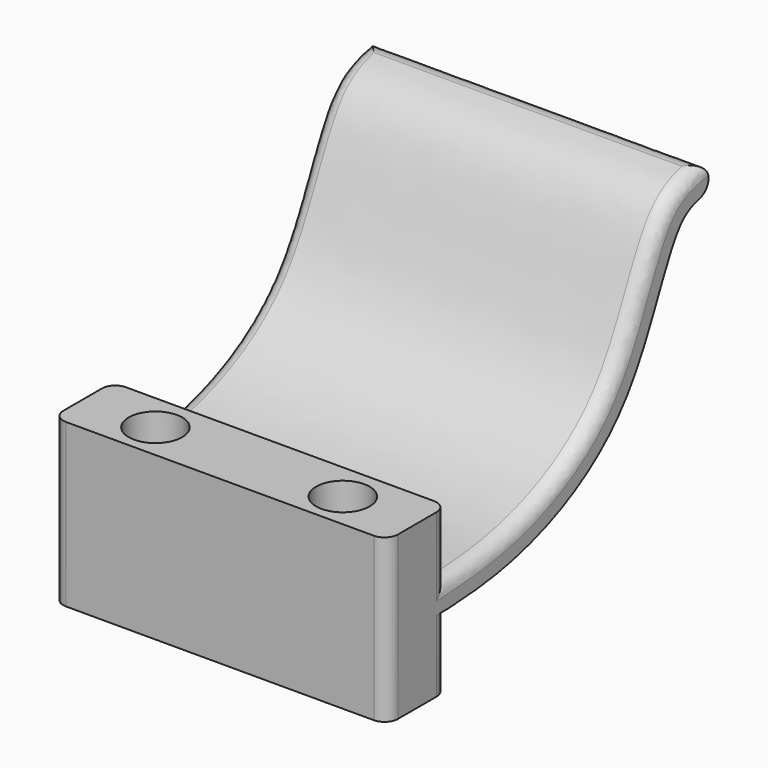
from build123d import *

# Parameters (mm, degrees)
F1_DEPTH       = 25
F3_DEPTH       = 25.001
F5_D           = 3
F5_DEPTH       = 12
F5_CBORE_D     = 4
F5_CBORE_DEPTH = 5
F5_TIP         = 0.9012909285
F6_R           = 1


# Not quite as in the source:
# - ends of sketch curves that miss each other by under 0.0002 mm in the source are joined
# - the dataset's text gives a spline's control points without its knots; the knots are read off the source's solid


with BuildPart() as f1:
    # F0 (on Top) → F1 (new body)
    with BuildSketch(Plane.XY):
        Polygon((12.5, 12.3358736806), (12.5, 15), (10.2798947338, 15), align=None)
        Polygon((12.5, 12.3358736806), (10.2798947338, 15), (7.0256240355, 15), (12.5, 8.4307488427), align=None)
        Polygon((12.5, 8.4307488427), (7.0256240355, 15), (3.7713532076, 15), (12.5, 4.5256238491), align=None)
        Polygon((12.5, 4.5256238491), (3.7713532076, 15), (0.5170825093, 15), (12.5, 0.6204990111), align=None)
        Polygon((12.5, 0.6204990111), (0.5170825093, 15), (-2.7371880471, 15), (12.5, -3.2846256565), align=None)
        Polygon((12.5, -3.2846256565), (-2.7371880471, 15), (-5.9914587454, 15), (12.5, -7.1897504944), align=None)
        Polygon((12.5, -7.1897504944), (-5.9914587454, 15), (-9.2457293017, 15), (12.5, -11.094875162), align=None)
        Polygon((12.5, -11.094875162), (-9.2457293017, 15), (-12.5, 15), (12.5, -15), align=None)
        Polygon((12.5, -15), (-12.5, 15), (-12.5, 11.094875162), (9.2457293017, -15), align=None)
        Polygon((5.9914586034, -15), (-12.5, 7.1897503241), (-12.5, 3.2846254861), (2.7371879051, -15), align=None)
        Polygon((-0.5170827932, -15), (-12.5, -0.6204993518), (-12.5, -4.5256241898), (-3.7713534915, -15), align=None)
        Polygon((-3.7713534915, -15), (-12.5, -4.5256241898), (-12.5, -8.4307490277), (-7.0256241898, -15), align=None)
        Polygon((-7.0256241898, -15), (-12.5, -8.4307490277), (-12.5, -15), align=None)
        Polygon((9.2457293017, -15), (-12.5, 11.094875162), (-12.5, 7.1897503241), (5.9914586034, -15), align=None)
        Polygon((2.7371879051, -15), (-12.5, 3.2846254861), (-12.5, -0.6204993518), (-0.5170827932, -15), align=None)
    extrude(amount=F1_DEPTH)

    # F2 (on face) → F3 (cut, through all)
    with BuildSketch(Plane(origin=(-12.5, 0, 0), x_dir=(0, -1, 0), z_dir=(-1, 0, 0))):
        with BuildLine():
            Line((15, 25), (-15, 25))
            add(Edge.make_bspline(
                [(-15, 25), (-13.5568248924, 24.7224313944), (-9.8278339599, 24.005227496), (-6.8122451266, 12.0375054671), (2.945956356, 7.7369731005), (7.4143120604, 7.46721459), (9.3878423795, 7.3480708525)],
                knots=[0, 0, 0, 0, 0.1895841201, 0.4898625685, 0.7746885533, 1, 1, 1, 1], degree=3))
            Line((9.3878423795, 7.3480708525), (9.3878423795, 12.1319638565))
            Line((9.3878423795, 12.1319638565), (15, 12.1319638565))
            Line((15, 12.1319638565), (15, 25))
        make_face()
        with BuildLine():
            Line((9.3878423795, 0), (9.3878423795, 5.3517055617))
            Line((9.3878423795, 5.3517055617), (9.2673200749, 5.3517055617))
            add(Edge.make_bspline(
                [(-15.0000575165, 22.9623060021), (-14.6750769086, 22.8974842127), (-14.1746868984, 22.789063183), (-13.5954276376, 22.6021711473), (-13.1732029655, 22.4090687875), (-12.867772976, 22.2113862359), (-12.6317224774, 22.0126010766), (-12.4567595118, 21.838250856), (-12.2734281701, 21.6221144569), (-12.0699637563, 21.3450122532), (-11.8562489345, 21.0163300592), (-11.5603798617, 20.5139838197), (-11.176165806, 19.7797133282), (-10.6958775361, 18.767836688), (-10.1906413822, 17.6609048928), (-9.6497850817, 16.4909565123), (-9.0591193515, 15.2873931399), (-8.401307085, 14.0777387133), (-7.7797470029, 13.0871929073), (-7.2259212866, 12.3190564954), (-6.6294247554, 11.5740230358), (-5.8330517423, 10.7238746842), (-4.469813467, 9.5191459149), (-2.6461329718, 8.2928627168), (-0.390600399, 7.2034186589), (1.8283532393, 6.4330776096), (3.8987281726, 5.9261842869), (6.4545278666, 5.5194639384), (8.1724298973, 5.4178050316), (9.2673200749, 5.3517055617)],
                knots=[0.0170522031, 0.0170522031, 0.0170522031, 0.0170522031, 0.0625, 0.09375, 0.125, 0.15625, 0.171875, 0.1875, 0.203125, 0.21875, 0.234375, 0.25, 0.28125, 0.3125, 0.34375, 0.375, 0.40625, 0.4375, 0.46875, 0.484375, 0.5, 0.53125, 0.5625, 0.625, 0.6875, 0.75, 0.8125, 0.875, 1, 1, 1, 1], degree=3))
            Line((-15.0000575165, 22.9623060021), (-15, 0))
            Line((-15, 0), (9.3878423795, 0))
        make_face()
    extrude(amount=-F3_DEPTH, mode=Mode.SUBTRACT)

    # F5
    with Locations(Plane.XY.offset(12.1319638565)):
        with Locations((-7, -12.2644081712), (7, -12.2644081712)):
            CounterBoreHole(F5_D / 2, F5_CBORE_D / 2, F5_CBORE_DEPTH, depth=F5_DEPTH)
            with Locations((0, 0, -(F5_DEPTH + F5_TIP / 2))):  # 118° drill point
                Cone(0, F5_D / 2, F5_TIP, mode=Mode.SUBTRACT)

    # F6
    f6_edges = [f1.edges().sort_by_distance(p)[0] for p in [
        (12.5, -15, 6.065982),
        (-12.5, -15, 6.065982),
        (12.5, 5.249403, 13.058777),
        (-12.5, 5.249403, 13.058777),
        (12.5, -9.387842, 9.740017),
        (-12.5, -9.387842, 9.740017),
        (0, 15, 25),
        (12.5, -9.387842, 2.675853),
        (-12.5, -9.387842, 2.675853),
        (0, 15, 22.962295),
    ]]
    fillet(f6_edges, radius=F6_R)


solid = f1.part
